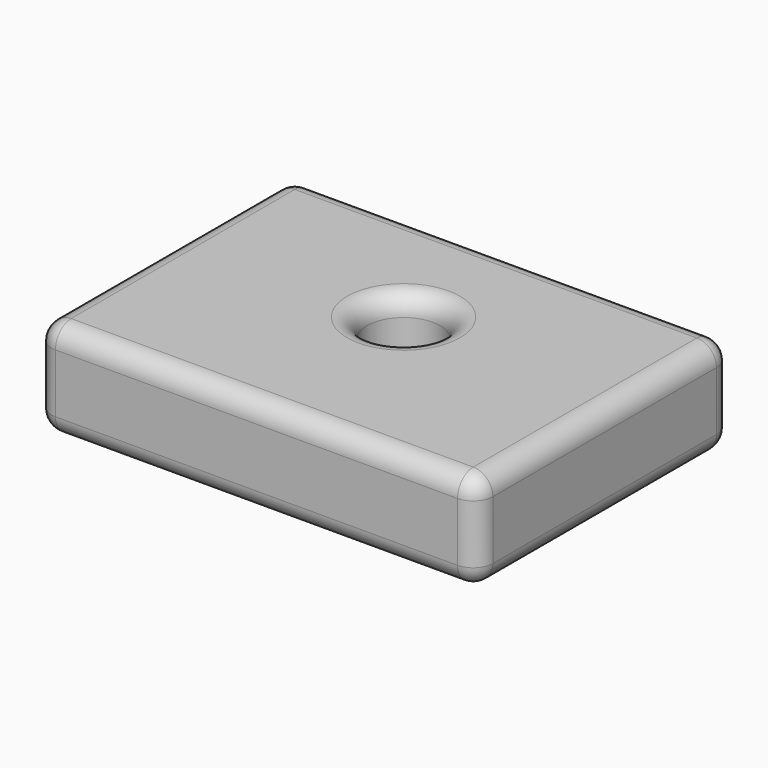
from build123d import *

# Parameters (mm, degrees)
F0_W         = 114.3
F0_H         = 82.55
F1_DEPTH     = 25.4
F2_R         = 9.525
F3_DEPTH     = 45.21898
F4_R         = 5.08
F5_T1_DEPTH  = 104.14
F5_T3_DEPTH  = 72.39
F5_S7_W      = 5.08
F5_S7_H      = 5.08
F5_T8_DEPTH  = 5.08
F5_S13_W     = 5.08
F5_S13_H     = 5.08
F5_T14_DEPTH = 5.08
F5_T20_ANGLE = 90


# Not quite as in the source:
# - a fillet or chamfer that OpenCascade refuses, or shapes differently, is made with other operations: its cross-section is extruded or revolved along the edge and cut away or added


with BuildPart() as f1:
    # F0 (on Top) → F1 (new body)
    with BuildSketch(Plane.XY):
        with Locations((-13.2126640528, 15.875)):
            Rectangle(F0_W, F0_H)
    extrude(amount=F1_DEPTH)

    # F2 (on face) → F3 (cut)
    with BuildSketch(Plane.XY.offset(25.4)):
        with Locations((-13.2126640528, 22.225)):
            Circle(F2_R)
    extrude(amount=-F3_DEPTH, mode=Mode.SUBTRACT)

    # F4
    f4_edges = [f1.edges().sort_by_distance(p)[0] for p in [
        (43.937336, 57.15, 12.7),
        (-70.362664, 57.15, 12.7),
        (43.937336, -25.4, 12.7),
        (-70.362664, -25.4, 12.7),
        (-13.212664, -25.4, 25.4),
        (-70.362664, 15.875, 25.4),
        (-70.362664, 15.875, 0),
        (43.937336, 15.875, 0),
        (-13.212664, -25.4, 0),
        (-13.212664, 57.15, 0),
        (-22.737664, 22.225, 0),
    ]]
    fillet(f4_edges, radius=F4_R)

    # F5: fillet of radius 5.08 on 2 edges, made by hand

    # F5_s2 → F5_t1 (cut)
    with BuildSketch(Plane.YZ.offset(-65.2826640528)):
        with BuildLine():
            ThreePointArc((52.07, 25.4), (55.6621024484, 23.9121024484), (57.15, 20.32))
            Line((57.15, 20.32), (57.15, 25.4))
            Line((57.15, 25.4), (52.07, 25.4))
        make_face()
    extrude(amount=F5_T1_DEPTH, mode=Mode.SUBTRACT)

    # F5_s4 → F5_t3 (cut)
    with BuildSketch(Plane.XZ.offset(-52.07)):
        with BuildLine():
            ThreePointArc((43.9373359472, 20.32), (42.4494383956, 23.9121024484), (38.8573359472, 25.4))
            Line((38.8573359472, 25.4), (43.9373359472, 25.4))
            Line((43.9373359472, 25.4), (43.9373359472, 20.32))
        make_face()
    extrude(amount=F5_T3_DEPTH, mode=Mode.SUBTRACT)


with BuildPart() as f5_tool6:
    # F5_s7 → F5_t8 (new body)
    with BuildSketch(Plane.XY.offset(20.32)):
        with Locations((-67.8226640528, 54.61)):
            Rectangle(F5_S7_W, F5_S7_H)
    extrude(amount=F5_T8_DEPTH)

    # F5_s9 → F5_t10 (revolve, cut)
    with BuildSketch(Plane(origin=(-65.2826640528, 52.07, 20.32), x_dir=(0.7071067812, -0.7071067812, 0), z_dir=(-0.7071067812, -0.7071067812, 0))):
        with BuildLine():
            ThreePointArc((0, -5.08), (5.08, 0), (0, 5.08))
            Line((0, 5.08), (0, -5.08))
        make_face()
    revolve(axis=Axis((-65.2826640528, 52.07, 20.32), (0, 0, 1)), mode=Mode.SUBTRACT)


with BuildPart() as f1_1:
    add(f1.part)

    # F5_t5: cut F5_tool6
    add(f5_tool6.part, mode=Mode.SUBTRACT)


with BuildPart() as f5_tool12:
    # F5_s13 → F5_t14 (new body)
    with BuildSketch(Plane.YZ.offset(38.8573359472)):
        with Locations((-22.86, 22.86)):
            Rectangle(F5_S13_W, F5_S13_H)
    extrude(amount=F5_T14_DEPTH)

    # F5_s15 → F5_t16 (revolve, cut)
    with BuildSketch(Plane(origin=(38.8573359472, -20.32, 20.32), x_dir=(0, 0.7071067812, -0.7071067812), z_dir=(0, -0.7071067812, -0.7071067812))):
        with BuildLine():
            ThreePointArc((0, -5.08), (5.08, 0), (0, 5.08))
            Line((0, 5.08), (0, -5.08))
        make_face()
    revolve(axis=Axis((38.8573359472, -20.32, 20.32), (1, 0, 0)), mode=Mode.SUBTRACT)


with BuildPart() as f1_2:
    add(f1_1.part)

    # F5_t11: cut F5_tool12
    add(f5_tool12.part, mode=Mode.SUBTRACT)

    # F5_s17 → F5_t18 (revolve, cut)
    with BuildSketch(Plane.XZ.offset(-22.225)):
        with BuildLine():
            ThreePointArc((1.3923359472, 25.4), (-2.1997665013, 23.9121024484), (-3.6876640528, 20.32))
            Line((-3.6876640528, 20.32), (-3.6876640528, 25.4))
            Line((-3.6876640528, 25.4), (1.3923359472, 25.4))
        make_face()
    revolve(axis=Axis((-13.2126640528, 22.225, 25.4), (0, 0, 1)), mode=Mode.SUBTRACT)

    # F5_s19 → F5_t20 (revolve, cut)
    with BuildSketch(Plane.XZ.offset(-52.07)):
        with BuildLine():
            ThreePointArc((38.8573359472, 25.4), (42.4494383956, 23.9121024484), (43.9373359472, 20.32))
            Line((43.9373359472, 20.32), (43.9373359472, 25.4))
            Line((43.9373359472, 25.4), (38.8573359472, 25.4))
        make_face()
    revolve(axis=Axis((38.8573359472, 52.07, 25.4), (0, 0, 1)), revolution_arc=F5_T20_ANGLE, mode=Mode.SUBTRACT)


solid = f1_2.part
